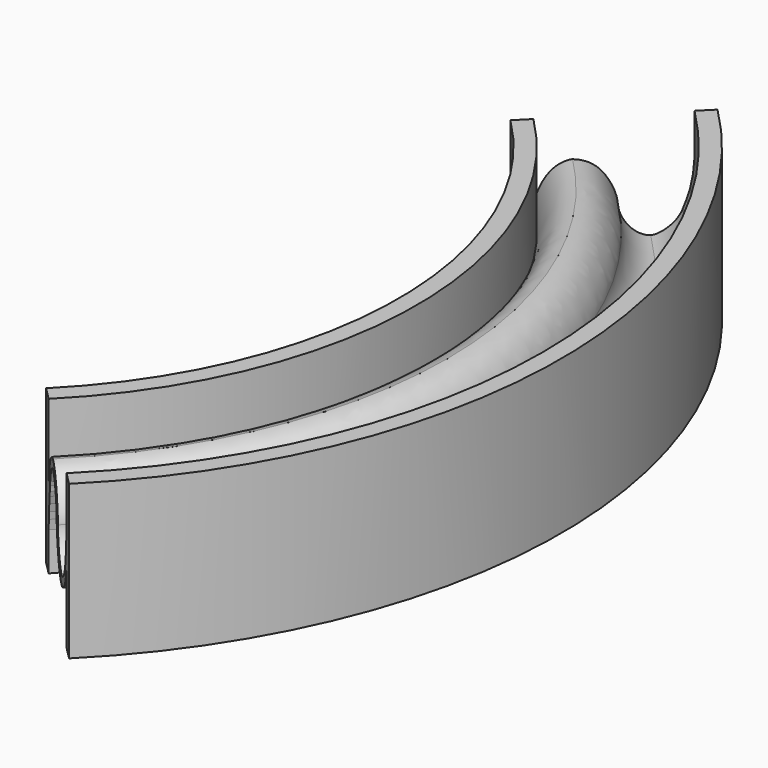
from build123d import *

# Parameters (mm, degrees)
F1_ANGLE_BACK = 45
F1_ANGLE      = 90


# Not quite as in the source:
# - ends of sketch curves that miss each other by under 0.0002 mm in the source are joined


with BuildPart() as f1:
    # F0 (on Front) → F1 (revolve)
    with BuildSketch(Plane.XZ, mode=Mode.PRIVATE) as f1_sk:
        Polygon((8, 4.2551231384), (8, 0), (9, 0), (9, 8.5), (8, 8.5), (8, 6.2273216248), align=None)
        Polygon((1, 2.124959883), (1, 4.2499679064), (1, 8.5), (0, 8.5), (0, 0), (1, 0), align=None)
        with BuildLine():
            add(Edge.make_bspline(
                [(1.6135353927, 4.7835650405), (1.6750901529, 4.970267715), (1.9288235062, 5.5585034544), (2.3534665623, 5.9191497273), (2.7, 5.9499679064)],
                knots=[0.2683438661, 0.2683438661, 0.2683438661, 0.2683438661, 0.5126436151, 1, 1, 1, 1], degree=3))
            Line((2.7, 5.9499679064), (2.7, 6.4499679064))
            add(Edge.make_bspline(
                [(1, 4.2499679064), (1.0015353048, 4.5626104683), (1.4551687546, 5.9442127178), (2.3433097433, 6.4271380926), (2.7, 6.4499679064)],
                knots=[0, 0, 0, 0, 0.5304369026, 1, 1, 1, 1], degree=3))
            Line((1, 4.2499679064), (1.4618344062, 4.2499679064))
            Line((1.4618344062, 4.2499679064), (1.5469024263, 4.5491884505))
            add(Edge.make_bspline(
                [(1.5469024263, 4.5491884505), (1.5645406816, 4.6235882391), (1.5868631876, 4.702665172), (1.6135353927, 4.7835650405)],
                knots=[0.1624866916, 0.1624866916, 0.1624866916, 0.1624866916, 0.2683438661, 0.2683438661, 0.2683438661, 0.2683438661], degree=3))
        make_face()
        with BuildLine():
            add(Edge.make_bspline(
                [(8, 4.2551231384), (7.9986488935, 3.9799898766), (7.7456702226, 2.8557466438), (6.505031952, 2.0758276235), (6.1, 2.0499037191)],
                knots=[0, 0, 0, 0, 0.4667977205, 1, 1, 1, 1], degree=3))
            Line((8, 4.2551231384), (8, 6.2273216248))
            Line((8, 6.2273216248), (7.9344944983, 5.4252070189))
            Line((7.9344944983, 5.4252070189), (7.801741117, 4.7100675088))
            Line((7.801741117, 4.7100675088), (7.6594823926, 4.2259131372))
            Line((7.6594823926, 4.2259131372), (7.5023478676, 3.7956271327))
            add(Edge.make_bspline(
                [(7.5023478676, 3.7956271327), (7.4950709382, 3.7744309229), (7.487268414, 3.753028112), (7.4789151485, 3.7314606417)],
                knots=[0.2362923479, 0.2362923479, 0.2362923479, 0.2362923479, 0.2672769863, 0.2672769863, 0.2672769863, 0.2672769863], degree=3))
            add(Edge.make_bspline(
                [(7.4789151485, 3.7314606417), (7.429977914, 3.6051085751), (7.1561404277, 3.07227024), (6.4919298971, 2.5847591313), (6.1, 2.5499037191)],
                knots=[0.2672769863, 0.2672769863, 0.2672769863, 0.2672769863, 0.4487991142, 1, 1, 1, 1], degree=3))
            add(Edge.make_bspline(
                [(6.1, 2.5499037191), (5.722922109, 2.560753403), (4.9562868612, 3.0652346955), (4.6679732537, 3.9028036589), (4.6499999995, 4.249903719)],
                knots=[0, 0, 0, 0, 0.5008610447, 1, 1, 1, 1], degree=3))
            add(Edge.make_bspline(
                [(2.7, 6.4499679064), (3.0971914861, 6.4159367347), (4.0379566942, 6.1199675516), (4.6572574431, 4.6342403799), (4.6499999995, 4.249903719)],
                knots=[0, 0, 0, 0, 0.4611151657, 0.9982015649, 0.9982015649, 0.9982015649, 0.9982015649], degree=3))
            Line((2.7, 6.4499679064), (2.7, 5.9499679064))
            add(Edge.make_bspline(
                [(2.7, 5.9499679064), (3.0770804596, 5.9391181486), (3.8437046032, 5.4345511486), (4.1320268683, 4.5970014065), (4.1499999995, 4.249903719)],
                knots=[0, 0, 0, 0, 0.5008644565, 1, 1, 1, 1], degree=3))
            add(Edge.make_bspline(
                [(4.3999999995, 3.3776864381), (4.2426068049, 3.7097412493), (4.1460321192, 4.0410870495), (4.1499999995, 4.249903719)],
                knots=[0.7063927669, 0.7063927669, 0.7063927669, 0.7063927669, 0.9982015652, 0.9982015652, 0.9982015652, 0.9982015652], degree=3))
            add(Edge.make_bspline(
                [(6.1, 2.0499037191), (5.7028107176, 2.0839347019), (5.0370554507, 2.2933169546), (4.5322969972, 3.0985774544), (4.3999999995, 3.3776864381)],
                knots=[0, 0, 0, 0, 0.4611126073, 0.7063927669, 0.7063927669, 0.7063927669, 0.7063927669], degree=3))
        make_face()
        with BuildLine():
            Line((1.5469024263, 4.5491884505), (1.6135353927, 4.7835650405))
            add(Edge.make_bspline(
                [(1.5469024263, 4.5491884505), (1.5645406816, 4.6235882391), (1.5868631876, 4.702665172), (1.6135353927, 4.7835650405)],
                knots=[0.1624866916, 0.1624866916, 0.1624866916, 0.1624866916, 0.2683438661, 0.2683438661, 0.2683438661, 0.2683438661], degree=3))
        make_face()
        Polygon((1.4618344062, 4.2499679064), (1, 4.2499679064), (1, 2.124959883), (1.0774135864, 2.6683010762), (1.144714681, 3.0744322246), (1.2561492896, 3.5201706593), (1.3731569326, 3.9380513733), align=None)
        with BuildLine():
            add(Edge.make_bspline(
                [(1.5, 4.2499679064), (1.5037909347, 4.3318066745), (1.5198283827, 4.4349876364), (1.5469024263, 4.5491884505)],
                knots=[0, 0, 0, 0, 0.1624866916, 0.1624866916, 0.1624866916, 0.1624866916], degree=3))
            Line((1.5469024263, 4.5491884505), (1.4618344062, 4.2499679064))
            Line((1.4618344062, 4.2499679064), (1.5, 4.2499679064))
        make_face()
    revolve(f1_sk.sketch.rotate(Axis((-22.7, 0, 2.7579944581), (0, 0, 1)), -F1_ANGLE_BACK), axis=Axis((-22.7, 0, 2.7579944581), (0, 0, 1)), revolution_arc=F1_ANGLE)


solid = f1.part
